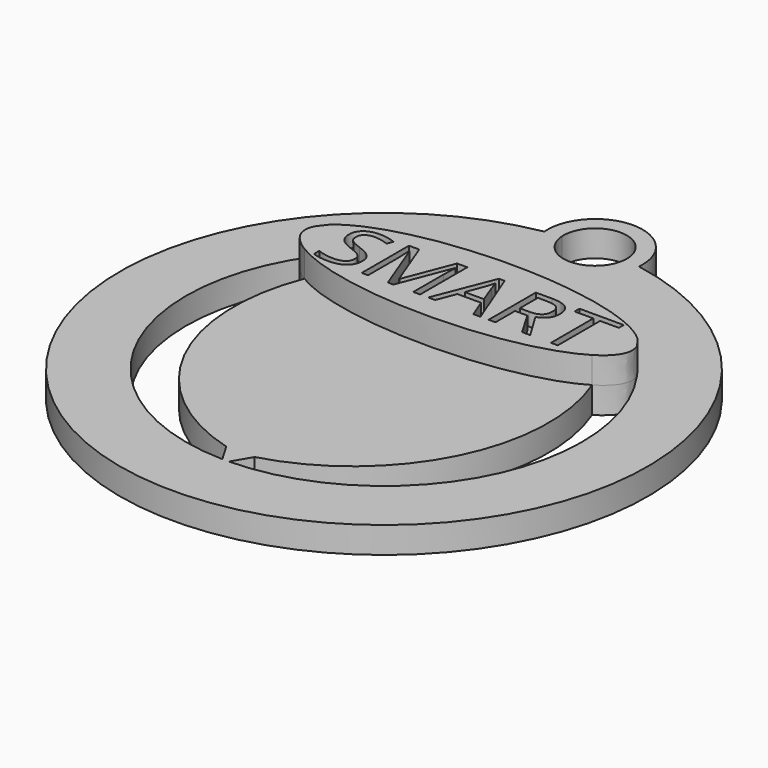
from build123d import *

# Parameters (mm, degrees)
F0_R          = 25.4
F0_R_2        = 19.05
F1_DEPTH      = 2.54
F3_DEPTH      = 2.54
F4_DEPTH      = 2.54
F4_DEPTH_BACK = 2.54
F5_TEXT_SIZE  = 7.9506125043
F6_DEPTH      = 1.27
F7_R          = 4.572
F8_DEPTH      = 2.54
F10_DEPTH     = 25.4


# Not quite as in the source:
# - Text() gives the source's letters only with a copy of the font that has no kerning and outlines rounded to 1/6400 em; it was checked with that copy


with BuildPart() as f1:
    # F0 (on Top) → F1 (new body)
    with BuildSketch(Plane.XY):
        Circle(F0_R)
        Circle(F0_R_2, mode=Mode.SUBTRACT)
    extrude(amount=F1_DEPTH)

    # F2 (on face) → F3 (join)
    with BuildSketch(Plane.XY.offset(2.54)):
        with BuildLine():
            add(Edge.make_bspline(
                [(1.6088081372, 15.4170151171), (0.2750903437, 15.4625914653), (-1.062595517, 15.4324889178)],
                knots=[1.4683430931, 1.4683430931, 1.4683430931, 1.6383984283, 1.6383984283, 1.6383984283], degree=2, weights=[1, 0.9963873252, 1]))
            Line((1.6088081372, 15.4170151171), (0.2812235516, 17.1259565513))
            Line((0.2812235516, 17.1259565513), (2.0530995219, 18.9390412205))
            ThreePointArc((2.0530995219, 18.9390412205), (1.0280478464, 19.0222400791), (0, 19.05))
            Line((0, 19.05), (-2.0841208904, 16.8224505556))
            Line((-2.0841208904, 16.8224505556), (-1.062595517, 15.4324889178))
        make_face()
        with BuildLine():
            add(Edge.make_bspline(
                [(-13.8442125171, 7.7336640097), (0, -0.7956921528), (13.8442125171, 7.7336640097)],
                knots=[3.6363263909, 3.6363263909, 3.6363263909, 5.7884515699, 5.7884515699, 5.7884515699], degree=2, weights=[1, 0.4747973316, 1]))
            ThreePointArc((-13.8442125171, 7.7336640097), (-13.1631256885, -7.5418639454), (-1.3617149089, -17.2646380961))
            Line((-1.3617149089, -17.2646380961), (-0.3145491167, -19.0474029425))
            ThreePointArc((-0.3145491167, -19.0474029425), (0, -19.05), (0.3145491167, -19.0474029425))
            Line((0.3145491167, -19.0474029425), (1.3617149089, -17.2646380961))
            ThreePointArc((1.3617149089, -17.2646380961), (13.1631256885, -7.5418639454), (13.8442125171, 7.7336640097))
        make_face()
    extrude(amount=-F3_DEPTH)

    # F2 (on face) → F4 (join, two sides)
    with BuildSketch(Plane.XY.offset(2.54)) as f4_sk:
        with BuildLine():
            add(Edge.make_bspline(
                [(14.8221063342, 11.9669404536), (11.4942351443, 15.0792062749), (1.6088081372, 15.4170151171)],
                knots=[0.3414766813, 0.3414766813, 0.3414766813, 1.4683430931, 1.4683430931, 1.4683430931], degree=2, weights=[1, 0.8454264498, 1]))
            add(Edge.make_bspline(
                [(1.6088081372, 15.4170151171), (0.2750903437, 15.4625914653), (-1.062595517, 15.4324889178)],
                knots=[1.4683430931, 1.4683430931, 1.4683430931, 1.6383984283, 1.6383984283, 1.6383984283], degree=2, weights=[1, 0.9963873252, 1]))
            add(Edge.make_bspline(
                [(-1.062595517, 15.4324889178), (-11.3643637539, 15.200663587), (-14.8221063342, 11.9669404536)],
                knots=[1.6383984283, 1.6383984283, 1.6383984283, 2.8001159722, 2.8001159722, 2.8001159722], degree=2, weights=[1, 0.8359917139, 1]))
            ThreePointArc((-14.8221063342, 11.9669404536), (-15.1943499794, 11.4906148097), (-15.5512925527, 11.0027178433))
            add(Edge.make_bspline(
                [(-15.5512925527, 11.0027178433), (-16.3431846368, 9.2732693302), (-13.8442125171, 7.7336640097)],
                knots=[2.9905619729, 2.9905619729, 2.9905619729, 3.6363263909, 3.6363263909, 3.6363263909], degree=2, weights=[1, 0.9483248301, 1]))
            add(Edge.make_bspline(
                [(-13.8442125171, 7.7336640097), (0, -0.7956921528), (13.8442125171, 7.7336640097)],
                knots=[3.6363263909, 3.6363263909, 3.6363263909, 5.7884515699, 5.7884515699, 5.7884515699], degree=2, weights=[1, 0.4747973316, 1]))
            add(Edge.make_bspline(
                [(13.8442125171, 7.7336640097), (15.7303586216, 8.8957100184), (15.7303586216, 10.2160740644)],
                knots=[5.7884515699, 5.7884515699, 5.7884515699, 6.2831853072, 6.2831853072, 6.2831853072], degree=2, weights=[1, 0.9695605092, 1]))
            add(Edge.make_bspline(
                [(15.7303586216, 10.2160740644), (15.7303586216, 10.6116474528), (15.5512925527, 11.0027178433)],
                knots=[0, 0, 0, 0.1510306807, 0.1510306807, 0.1510306807], degree=2, weights=[1, 0.9971500714, 1]))
            ThreePointArc((15.5512925527, 11.0027178433), (15.1943499794, 11.4906148097), (14.8221063342, 11.9669404536))
        make_face()
    extrude(amount=F4_DEPTH)
    extrude(f4_sk.sketch, amount=-F4_DEPTH_BACK)

    # F5 (on face) → F6 (cut)
    with BuildSketch(Plane.XY.offset(5.08)):
        with Locations((-13.1638539691, 7.3538535628)):
            Text('SMART', F5_TEXT_SIZE, font='Open Sans', text_align=(TextAlign.LEFT, TextAlign.BOTTOM))
    extrude(amount=-F6_DEPTH, mode=Mode.SUBTRACT)

    # F7 (on face) → F8 (join)
    with BuildSketch(Plane.XY.offset(2.54)):
        with Locations((0, 25.4028141499)):
            Circle(F7_R)
    extrude(amount=-F8_DEPTH)

    # F9 (on face) → F10 (cut)
    with BuildSketch(Plane.XY.offset(2.54)):
        with BuildLine():
            ThreePointArc((3.0422713031, 25.2171486358), (0, 25.4), (-3.0422713031, 25.2171486358))
            ThreePointArc((-3.0422713031, 25.2171486358), (0, 22.3559354622), (3.0422713031, 25.2171486358))
        make_face()
        with BuildLine():
            ThreePointArc((3.0422713031, 25.2171486358), (3.0465674891, 25.310498135), (3.048, 25.4039354622))
            ThreePointArc((3.048, 25.4039354622), (-0.0934373273, 28.4505029514), (-3.0422713031, 25.2171486358))
            ThreePointArc((-3.0422713031, 25.2171486358), (0, 25.4), (3.0422713031, 25.2171486358))
        make_face()
    extrude(amount=-F10_DEPTH, mode=Mode.SUBTRACT)


solid = f1.part
